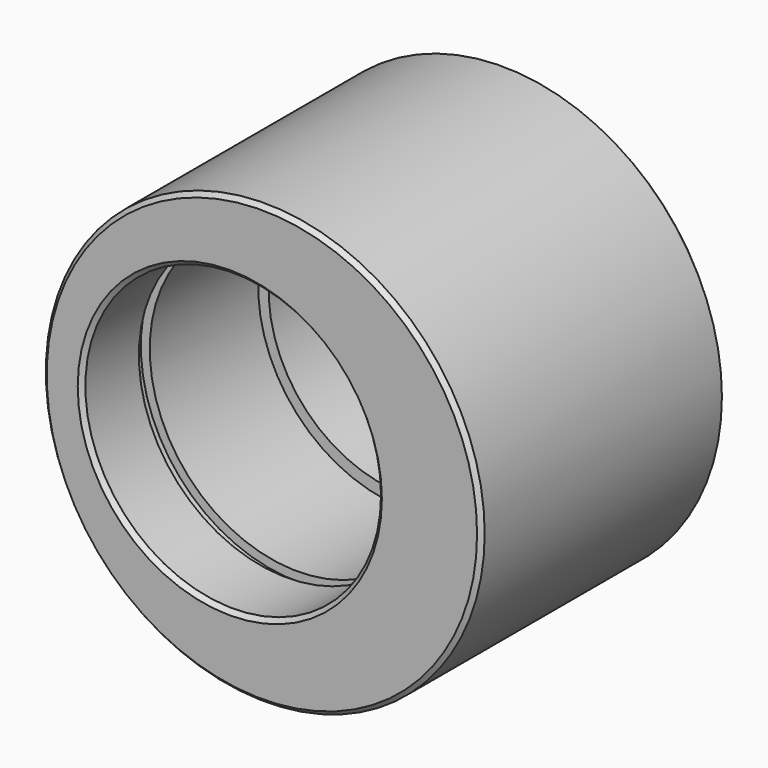
from build123d import *

# Parameters (mm, degrees)
F0_R     = 25.9
F0_R_2   = 16
F1_DEPTH = 10
F3_R     = 25.9
F3_R_2   = 17.45
F4_DEPTH = 16
F5_R     = 25.9
F5_R_2   = 18.5
F6_DEPTH = 1.6
F7_R     = 25.9
F7_R_2   = 18.5
F7_R_3   = 17.45
F8_DEPTH = 8.4
F9_SIZE  = 0.5
F10_SIZE = 0.5
F11_SIZE = 0.5


# Not quite as in the source:
# - a feature names something its author has since deleted; it is built from what else it names


with BuildPart() as f1:
    # F0 (on Front) → F1 (new body)
    with BuildSketch(Plane.XZ):
        Circle(F0_R)
        with Locations((-4, 0)):
            Circle(F0_R_2, mode=Mode.SUBTRACT)
    extrude(amount=F1_DEPTH)

    # F3 (on face) → F4 (join)
    with BuildSketch(Plane.XZ.offset(10)):
        Circle(F3_R)
        with Locations((-3.7866821816, 0)):
            Circle(F3_R_2, mode=Mode.SUBTRACT)
    extrude(amount=F4_DEPTH)

    # F5 (on face) → F6 (join)
    with BuildSketch(Plane.XZ.offset(26)):
        Circle(F5_R)
        with Locations((-3.7866821816, 0)):
            Circle(F5_R_2, mode=Mode.SUBTRACT)
    extrude(amount=F6_DEPTH)

    # F7 (on face) → F8 (join)
    with BuildSketch(Plane.XZ.offset(27.6)):
        Circle(F7_R)
        with Locations((-3.7866821816, 0)):
            Circle(F7_R_2, mode=Mode.SUBTRACT)
        with Locations((-3.7866821816, 0)):
            Circle(F7_R_2)
        with Locations((-3.7866821816, 0)):
            Circle(F7_R_3, mode=Mode.SUBTRACT)
    extrude(amount=F8_DEPTH)

    # F9
    f9_edges = [f1.edges().sort_by_distance(p)[0] for p in [
        (-25.9, 0, 0),
    ]]
    chamfer(f9_edges, length=F9_SIZE)

    # F10
    f10_edges = [f1.edges().sort_by_distance(p)[0] for p in [
        (-25.9, -36, 0),
    ]]
    chamfer(f10_edges, length=F10_SIZE)

    # F11
    f11_edges = [f1.edges().sort_by_distance(p)[0] for p in [
        (-21.236682, -36, 0),
    ]]
    chamfer(f11_edges, length=F11_SIZE)


solid = f1.part
